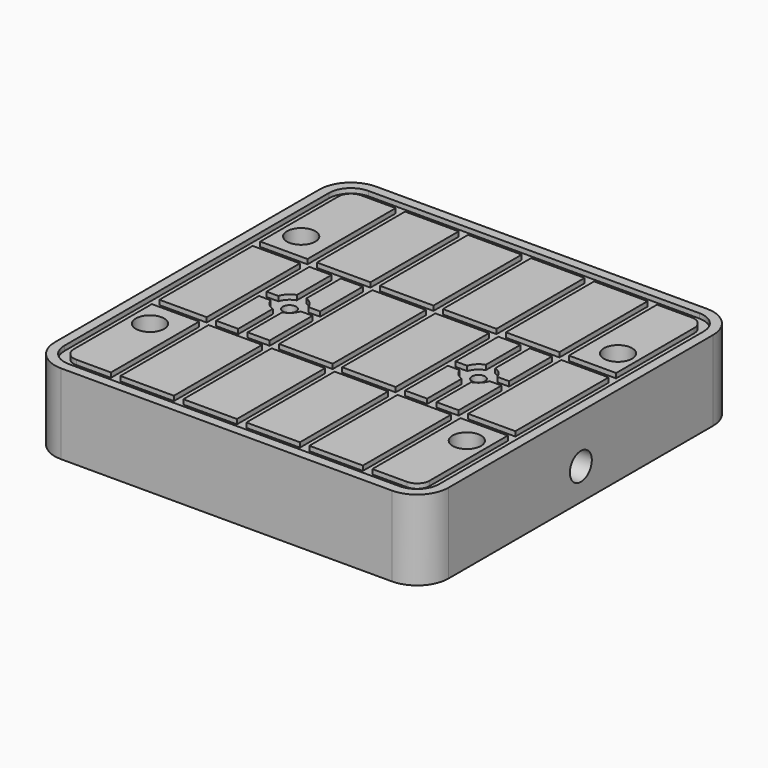
from build123d import *

# Parameters (mm, degrees)
F0_R      = 2.6
F1_DEPTH  = 9
F3_DEPTH  = 16.4
F4_R      = 2.5
F5_DEPTH  = 125.001
F4_R_2    = 4.35
F6_DEPTH  = 10
F7_DEPTH  = 25
F8_R      = 4.5
F9_DEPTH  = 15
F11_R     = 2.6
F12_DEPTH = 25
F13_W     = 113
F13_H     = 3
F14_DEPTH = 1.5
F15_W     = 3
F15_H     = 35
F15_H_2   = 78
F16_DEPTH = 1.5
F17_R     = 2.1
F18_DEPTH = 16
F19_R     = 5
F20_DEPTH = 1.5
F21_W     = 3
F21_H     = 3
F22_DEPTH = 1.5
F23_R     = 4.35
F23_R_2   = 2.5
F24_DEPTH = 10


# Not quite as in the source:
# - a feature names something its author has since deleted; it is built from what else it names


with BuildPart() as f1:
    # F0 (on Top) → F1 (new body)
    with BuildSketch(Plane.XY):
        with BuildLine():
            Line((-57.5, -72.5), (57.5, -72.5))
            ThreePointArc((57.5, -72.5), (61.0355339059, -71.0355339059), (62.5, -67.5))
            Line((62.5, -67.5), (62.5, 67.5))
            ThreePointArc((62.5, 67.5), (61.0355339059, 71.0355339059), (57.5, 72.5))
            Line((57.5, 72.5), (-57.5, 72.5))
            ThreePointArc((-57.5, 72.5), (-61.0355339059, 71.0355339059), (-62.5, 67.5))
            Line((-62.5, 67.5), (-62.5, -67.5))
            ThreePointArc((-62.5, -67.5), (-61.0355339059, -71.0355339059), (-57.5, -72.5))
        make_face()
        with Locations((-30, -67.5)):
            Circle(F0_R, mode=Mode.SUBTRACT)
        with Locations((30, -67.5)):
            Circle(F0_R, mode=Mode.SUBTRACT)
        with Locations((-30, 67.5)):
            Circle(F0_R, mode=Mode.SUBTRACT)
        with Locations((30, 67.5)):
            Circle(F0_R, mode=Mode.SUBTRACT)
    extrude(amount=F1_DEPTH)

    # F2 (on face) → F3 (join)
    with BuildSketch(Plane.XY.offset(9)):
        with BuildLine():
            Line((-52.5, -62.5), (52.5, -62.5))
            ThreePointArc((52.5, -62.5), (59.5710678119, -59.5710678119), (62.5, -52.5))
            Line((62.5, -52.5), (62.5, 52.5))
            ThreePointArc((62.5, 52.5), (59.5710678119, 59.5710678119), (52.5, 62.5))
            Line((52.5, 62.5), (-52.5, 62.5))
            ThreePointArc((-52.5, 62.5), (-59.5710678119, 59.5710678119), (-62.5, 52.5))
            Line((-62.5, 52.5), (-62.5, -52.5))
            ThreePointArc((-62.5, -52.5), (-59.5710678119, -59.5710678119), (-52.5, -62.5))
        make_face()
    extrude(amount=F3_DEPTH)

    # F4 (on face) → F5 (cut, through all)
    with BuildSketch(Plane.YZ.offset(62.5)):
        with Locations((0, 10)):
            Circle(F4_R)
    extrude(amount=-F5_DEPTH, mode=Mode.SUBTRACT)

    # F4 (on face) → F6 (cut)
    with BuildSketch(Plane.YZ.offset(62.5)):
        with Locations((0, 10)):
            Circle(F4_R_2)
        with Locations((0, 10)):
            Circle(F4_R, mode=Mode.SUBTRACT)
    extrude(amount=-F6_DEPTH, mode=Mode.SUBTRACT)

    # F7 (cut): faces of the model
    f7_faces = [f1.faces().sort_by_distance(p)[0] for p in [
        (0, -67.2159519927, 9),
        (0, 67.2159519927, 9),
    ]]
    extrude(f7_faces, amount=-F7_DEPTH, mode=Mode.SUBTRACT)

    # F8 (on face) → F9 (cut)
    with BuildSketch(Plane.XY.offset(25.4)):
        with Locations((-50.3, 30)):
            Circle(F8_R)
        with Locations((50.3, 30)):
            Circle(F8_R)
        with Locations((-50.3, -30)):
            Circle(F8_R)
        with Locations((50.3, -30)):
            Circle(F8_R)
    extrude(amount=-F9_DEPTH, mode=Mode.SUBTRACT)

    # F11 (on face) → F12 (cut)
    with BuildSketch(Plane.XY.offset(25.4)):
        with Locations((-50.3, 30)):
            Circle(F11_R)
        with Locations((50.3, 30)):
            Circle(F11_R)
        with Locations((50.3, -30)):
            Circle(F11_R)
        with Locations((-50.3, -30)):
            Circle(F11_R)
    extrude(amount=-F12_DEPTH, mode=Mode.SUBTRACT)

    # F13 (on face) → F14 (cut)
    with BuildSketch(Plane.XY.offset(25.4)):
        with BuildLine():
            Line((59.5, -52.5), (59.5, 52.5))
            ThreePointArc((59.5, 52.5), (57.4497474683, 57.4497474683), (52.5, 59.5))
            Line((52.5, 59.5), (-52.5, 59.5))
            ThreePointArc((-52.5, 59.5), (-57.4497474683, 57.4497474683), (-59.5, 52.5))
            Line((-59.5, 52.5), (-59.5, -52.5))
            ThreePointArc((-59.5, -52.5), (-57.4497474683, -57.4497474683), (-52.5, -59.5))
            Line((-52.5, -59.5), (52.5, -59.5))
            ThreePointArc((52.5, -59.5), (57.4497474683, -57.4497474683), (59.5, -52.5))
        make_face()
        with BuildLine():
            Line((-52.5, 56.5), (52.5, 56.5))
            ThreePointArc((52.5, 56.5), (55.3284271247, 55.3284271247), (56.5, 52.5))
            Line((56.5, 52.5), (56.5, 21.5))
            Line((56.5, 21.5), (56.5, 18.5))
            Line((56.5, 18.5), (56.5, -18.5))
            Line((56.5, -18.5), (56.5, -21.5))
            Line((56.5, -21.5), (56.5, -52.5))
            ThreePointArc((56.5, -52.5), (55.3284271247, -55.3284271247), (52.5, -56.5))
            Line((52.5, -56.5), (-52.5, -56.5))
            ThreePointArc((-52.5, -56.5), (-55.3284271247, -55.3284271247), (-56.5, -52.5))
            Line((-56.5, -52.5), (-56.5, -21.5))
            Line((-56.5, -21.5), (-56.5, -18.5))
            Line((-56.5, -18.5), (-56.5, 18.5))
            Line((-56.5, 18.5), (-56.5, 21.5))
            Line((-56.5, 21.5), (-56.5, 52.5))
            ThreePointArc((-56.5, 52.5), (-55.3284271247, 55.3284271247), (-52.5, 56.5))
        make_face(mode=Mode.SUBTRACT)
        with Locations((0, 20)):
            Rectangle(F13_W, F13_H)
        with Locations((0, -20)):
            Rectangle(F13_W, F13_H)
    extrude(amount=-F14_DEPTH, mode=Mode.SUBTRACT)

    # F15 (on face) → F16 (cut)
    with BuildSketch(Plane.XY.offset(25.4)):
        with Locations((-40, 39)):
            Rectangle(F15_W, F15_H)
        with Locations((-40, -17.5)):
            Rectangle(F15_W, F15_H_2)
        with Locations((-20, 39)):
            Rectangle(F15_W, F15_H)
        with Locations((-20, -17.5)):
            Rectangle(F15_W, F15_H_2)
        with Locations((0, 39)):
            Rectangle(F15_W, F15_H)
        with Locations((0, -17.5)):
            Rectangle(F15_W, F15_H_2)
        with Locations((20, -17.5)):
            Rectangle(F15_W, F15_H_2)
        with Locations((20, 39)):
            Rectangle(F15_W, F15_H)
        with Locations((40, 39)):
            Rectangle(F15_W, F15_H)
        with Locations((40, -17.5)):
            Rectangle(F15_W, F15_H_2)
    extrude(amount=-F16_DEPTH, mode=Mode.SUBTRACT)

    # F17 (on face) → F18 (cut)
    with BuildSketch(Plane.XY.offset(25.4)):
        with Locations((-30, 0)):
            Circle(F17_R)
        with Locations((30, 0)):
            Circle(F17_R)
    extrude(amount=-F18_DEPTH, mode=Mode.SUBTRACT)

    # F19 (on face) → F20 (cut)
    with BuildSketch(Plane.XY.offset(25.4)):
        with Locations((-30, 0)):
            Circle(F19_R)
        with Locations((30, 0)):
            Circle(F19_R)
    extrude(amount=-F20_DEPTH, mode=Mode.SUBTRACT)

    # F21 (on face) → F22 (cut)
    with BuildSketch(Plane.XY.offset(25.4)):
        with BuildLine():
            ThreePointArc((31.5, 18.5), (30, 20), (28.5, 18.5))
            Line((28.5, 18.5), (28.5, 1.5))
            Line((28.5, 1.5), (31.5, 1.5))
            Line((31.5, 1.5), (31.5, 18.5))
        make_face()
        with Locations((30, 0)):
            Rectangle(F21_W, F21_H)
        with BuildLine():
            Line((28.5, -1.5), (28.5, 1.5))
            Line((28.5, 1.5), (21.5, 1.5))
            ThreePointArc((21.5, 1.5), (20, 0), (21.5, -1.5))
            Line((21.5, -1.5), (28.5, -1.5))
        make_face()
        with BuildLine():
            Line((38.5, 1.5), (31.5, 1.5))
            Line((31.5, 1.5), (31.5, -1.5))
            Line((31.5, -1.5), (38.5, -1.5))
            ThreePointArc((38.5, -1.5), (40, 0), (38.5, 1.5))
        make_face()
        with BuildLine():
            Line((31.5, -1.5), (28.5, -1.5))
            Line((28.5, -1.5), (28.5, -18.5))
            ThreePointArc((28.5, -18.5), (30, -20), (31.5, -18.5))
            Line((31.5, -18.5), (31.5, -1.5))
        make_face()
        with BuildLine():
            ThreePointArc((-38.5, 1.5), (-40, 0), (-38.5, -1.5))
            Line((-38.5, -1.5), (-31.5, -1.5))
            Line((-31.5, -1.5), (-31.5, 1.5))
            Line((-31.5, 1.5), (-38.5, 1.5))
        make_face()
        with Locations((-30, 0)):
            Rectangle(F21_W, F21_H)
        with BuildLine():
            Line((-28.5, -1.5), (-31.5, -1.5))
            Line((-31.5, -1.5), (-31.5, -18.5))
            ThreePointArc((-31.5, -18.5), (-30, -20), (-28.5, -18.5))
            Line((-28.5, -18.5), (-28.5, -1.5))
        make_face()
        with BuildLine():
            Line((-31.5, 18.5), (-31.5, 1.5))
            Line((-31.5, 1.5), (-28.5, 1.5))
            Line((-28.5, 1.5), (-28.5, 18.5))
            ThreePointArc((-28.5, 18.5), (-30, 20), (-31.5, 18.5))
        make_face()
        with BuildLine():
            Line((-28.5, 1.5), (-28.5, -1.5))
            Line((-28.5, -1.5), (-21.5, -1.5))
            ThreePointArc((-21.5, -1.5), (-20, 0), (-21.5, 1.5))
            Line((-21.5, 1.5), (-28.5, 1.5))
        make_face()
    extrude(amount=-F22_DEPTH, mode=Mode.SUBTRACT)

    # F23 (on face) → F24 (cut)
    with BuildSketch(Plane(origin=(-62.5, 0, 0), x_dir=(0, -1, 0), z_dir=(-1, 0, 0))):
        with Locations((0, 10)):
            Circle(F23_R)
        with Locations((0, 10)):
            Circle(F23_R_2, mode=Mode.SUBTRACT)
    extrude(amount=-F24_DEPTH, mode=Mode.SUBTRACT)


solid = f1.part
